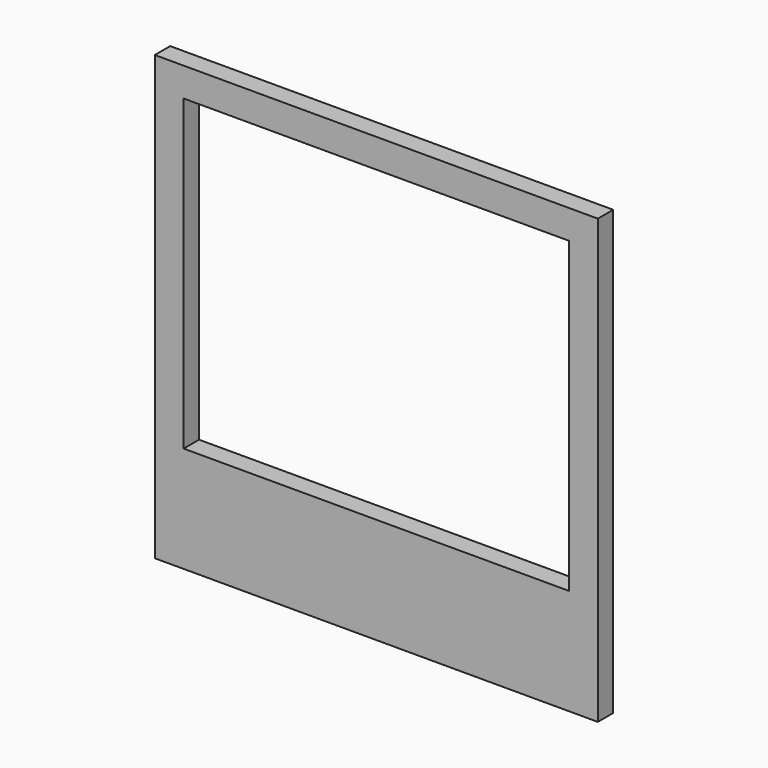
from build123d import *

# Parameters (mm, degrees)
F0_W     = 230
F0_H     = 40
F0_H_2   = 190
F0_W_2   = 200
F0_H_3   = 159.9997122972
F1_DEPTH = 10


# Not quite as in the source:
# - a feature names something its author has since deleted; it is built from what else it names


with BuildPart() as f1:
    # F0 (on Front) → F1 (new body)
    with BuildSketch(Plane.XZ):
        with Locations((0.0107780099, -35.0002877028)):
            Rectangle(F0_W, F0_H)
        with Locations((0.0107780099, 79.9997122972)):
            Rectangle(F0_W, F0_H_2)
        with Locations((0.0107780099, 79.9998561486)):
            Rectangle(F0_W_2, F0_H_3, mode=Mode.SUBTRACT)
    extrude(amount=F1_DEPTH)


solid = f1.part
